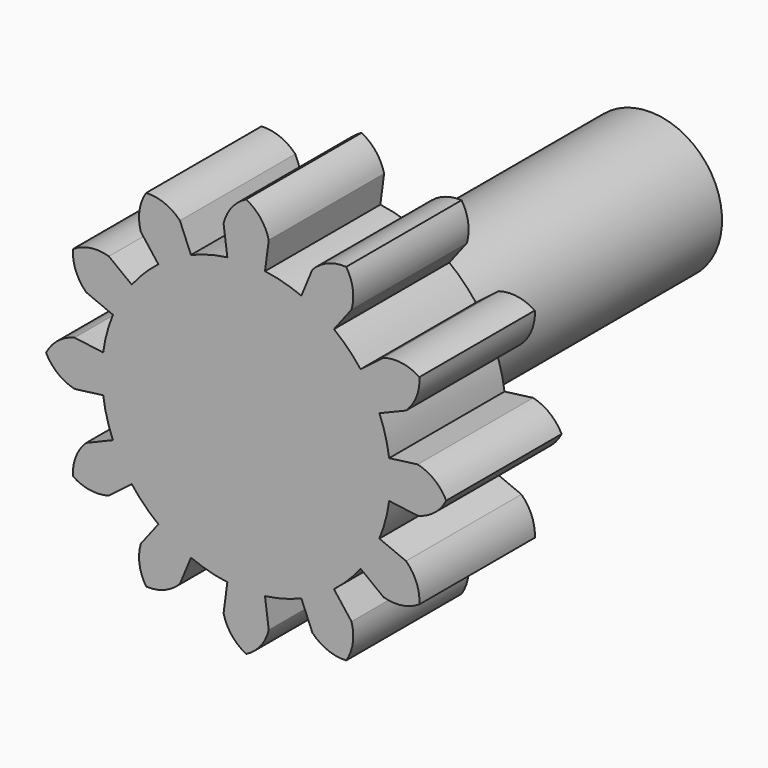
from build123d import *

# Parameters (mm, degrees)
F2_DEPTH        = 10
F2_COPIES_COUNT = 12
F4_R            = 10
F5_DEPTH        = 50


# Not quite as in the source:
# - a feature of the source that left no trace in its solid (it failed there, or was rolled back) is left out
# - a pattern or mirror of a feature is missing from the dataset's text; its kind, count and spacing are read off the source's solid


with BuildPart() as f2:
    # F1 (on Front) → F2 (new body, symmetric)
    with BuildSketch(Plane.XZ):
        with BuildLine():
            ThreePointArc((-2.6105238444, 19.8288972275), (-13.186916302, -15.0367961496), (20, 0))
            ThreePointArc((20, 0), (15.0367961496, 13.186916302), (2.6105238444, 19.8288972275))
            ThreePointArc((2.6105238444, 19.8288972275), (0, 20), (-2.6105238444, 19.8288972275))
        make_face()
        with BuildLine():
            ThreePointArc((-2.6105238444, 19.8288972275), (0, 20), (2.6105238444, 19.8288972275))
            Line((2.6105238444, 19.8288972275), (3.1326286133, 23.794676673))
            ThreePointArc((3.1326286133, 23.794676673), (2.0019466325, 26.1165955987), (0, 27.7481466766))
            ThreePointArc((0, 27.7481466766), (-2.0019466325, 26.1165955987), (-3.1326286133, 23.794676673))
            Line((-3.1326286133, 23.794676673), (-2.6105238444, 19.8288972275))
        make_face()
    extrude(amount=F2_DEPTH, both=True)

    # F2_copies: F2 ×12 about axis
    f2_copies_axis = Axis((0, 0, 0), (0, 1, 0))


with BuildPart() as f2_1:
    add(f2.part)
    for i in range(1, F2_COPIES_COUNT):
        add(f2.part.rotate(f2_copies_axis, i * 360 / F2_COPIES_COUNT))

    # F4 (on face) → F5 (join)
    with BuildSketch(Plane(origin=(0, 10, 0), x_dir=(-1, 0, 0), z_dir=(0, 1, 0))):
        Circle(F4_R)
    extrude(amount=F5_DEPTH)


solid = f2_1.part
